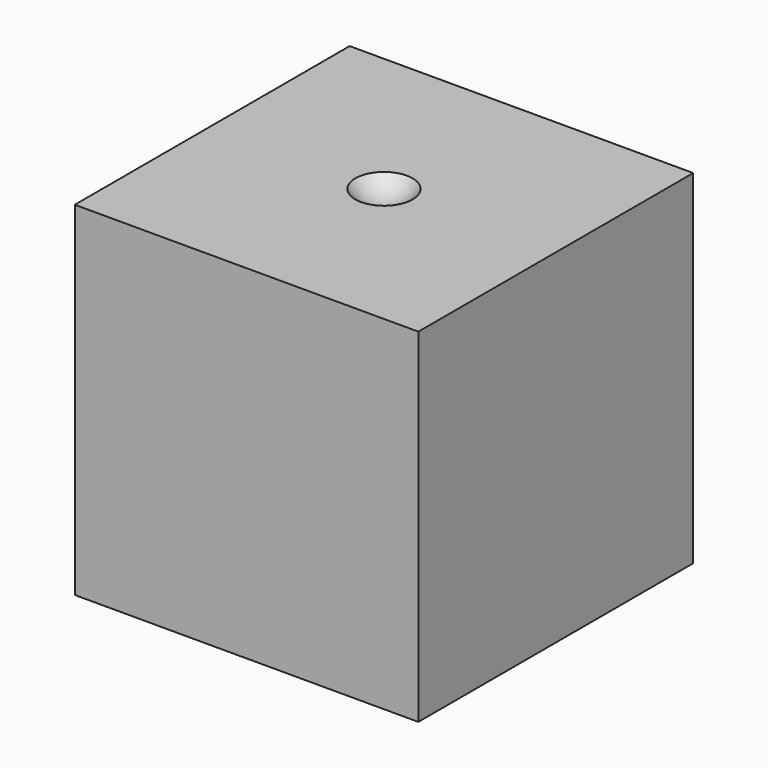
from build123d import *

# Parameters (mm, degrees)
F0_W     = 152.4
F0_H     = 152.4
F1_DEPTH = 152.4
F2_R     = 12.7
F3_DEPTH = 6.35
F5_R     = 12.7
F6_DEPTH = 6.35
F8_R     = 12.7
F9_DEPTH = 6.35


# Not quite as in the source:
# - a fillet or chamfer that OpenCascade refuses, or shapes differently, is made with other operations: its cross-section is extruded or revolved along the edge and cut away or added


with BuildPart() as f1:
    # F0 (on Front) → F1 (new body)
    with BuildSketch(Plane.XZ):
        Rectangle(F0_W, F0_H)
    extrude(amount=F1_DEPTH)

    # F2 (on face) → F3 (cut)
    with BuildSketch(Plane.XY.offset(76.2)):
        with Locations((0, -76.2)):
            Circle(F2_R)
    extrude(amount=-F3_DEPTH, mode=Mode.SUBTRACT)

    # F4: fillet of radius 15.8496 on 1 edges, made by hand

    # F4_s1 → F4_t2 (revolve)
    with BuildSketch(Plane.XZ.offset(76.2)):
        with BuildLine():
            ThreePointArc((12.7, 76.2), (7.1065402986, 71.5261268844), (0.0127063564, 69.85))
            Line((0.0127063564, 69.85), (12.7, 69.85))
            Line((12.7, 69.85), (12.7, 76.2))
        make_face()
    revolve(axis=Axis((0, -76.2, 69.85), (0, 0, 1)))

    # F5 (on face) → F6 (cut)
    with BuildSketch(Plane(origin=(0, 0, -76.2), x_dir=(1, 0, 0), z_dir=(0, 0, -1))):
        with Locations((50.8, 19.05)):
            Circle(F5_R)
        with Locations((50.8, 76.2)):
            Circle(F5_R)
        with Locations((-50.8, 19.05)):
            Circle(F5_R)
        with Locations((-50.8, 76.2)):
            Circle(F5_R)
        with Locations((-50.8, 133.35)):
            Circle(F5_R)
        with Locations((50.8, 133.35)):
            Circle(F5_R)
    extrude(amount=-F6_DEPTH, mode=Mode.SUBTRACT)

    # F7: fillet of radius 15.8496 on 6 edges, made by hand

    # F7_s1 → F7_t2 (revolve)
    with BuildSketch(Plane.XZ.offset(19.05)):
        with BuildLine():
            ThreePointArc((63.5, -76.2), (57.9065402986, -71.5261268844), (50.8127063564, -69.85))
            Line((50.8127063564, -69.85), (63.5, -69.85))
            Line((63.5, -69.85), (63.5, -76.2))
        make_face()
    revolve(axis=Axis((50.8, -19.05, -69.85), (0, 0, -1)))

    # F7_s3 → F7_t4 (revolve)
    with BuildSketch(Plane.XZ.offset(76.2)):
        with BuildLine():
            ThreePointArc((63.5, -76.2), (57.9065402986, -71.5261268844), (50.8127063564, -69.85))
            Line((50.8127063564, -69.85), (63.5, -69.85))
            Line((63.5, -69.85), (63.5, -76.2))
        make_face()
    revolve(axis=Axis((50.8, -76.2, -69.85), (0, 0, -1)))

    # F7_s5 → F7_t6 (revolve)
    with BuildSketch(Plane.XZ.offset(133.35)):
        with BuildLine():
            ThreePointArc((63.5, -76.2), (57.9065402986, -71.5261268844), (50.8127063564, -69.85))
            Line((50.8127063564, -69.85), (63.5, -69.85))
            Line((63.5, -69.85), (63.5, -76.2))
        make_face()
    revolve(axis=Axis((50.8, -133.35, -69.85), (0, 0, -1)))

    # F7_s7 → F7_t8 (revolve)
    with BuildSketch(Plane.XZ.offset(19.05)):
        with BuildLine():
            ThreePointArc((-38.1, -76.2), (-43.6934597014, -71.5261268844), (-50.7872936436, -69.85))
            Line((-50.7872936436, -69.85), (-38.1, -69.85))
            Line((-38.1, -69.85), (-38.1, -76.2))
        make_face()
    revolve(axis=Axis((-50.8, -19.05, -69.85), (0, 0, -1)))

    # F7_s9 → F7_t10 (revolve)
    with BuildSketch(Plane.XZ.offset(76.2)):
        with BuildLine():
            ThreePointArc((-38.1, -76.2), (-43.6934597014, -71.5261268844), (-50.7872936436, -69.85))
            Line((-50.7872936436, -69.85), (-38.1, -69.85))
            Line((-38.1, -69.85), (-38.1, -76.2))
        make_face()
    revolve(axis=Axis((-50.8, -76.2, -69.85), (0, 0, -1)))

    # F7_s11 → F7_t12 (revolve)
    with BuildSketch(Plane.XZ.offset(133.35)):
        with BuildLine():
            ThreePointArc((-38.1, -76.2), (-43.6934597014, -71.5261268844), (-50.7872936436, -69.85))
            Line((-50.7872936436, -69.85), (-38.1, -69.85))
            Line((-38.1, -69.85), (-38.1, -76.2))
        make_face()
    revolve(axis=Axis((-50.8, -133.35, -69.85), (0, 0, -1)))

    # F8 (on face) → F9 (join)
    with BuildSketch(Plane(origin=(0, 0, 0), x_dir=(-1, 0, 0), z_dir=(0, 1, 0))):
        with Locations((50.8, -57.15)):
            Circle(F8_R)
        with Locations((-50.8, -57.15)):
            Circle(F8_R)
        with Locations((-50.8, 57.15)):
            Circle(F8_R)
        with Locations((50.8, 57.15)):
            Circle(F8_R)
    extrude(amount=-F9_DEPTH)


solid = f1.part
